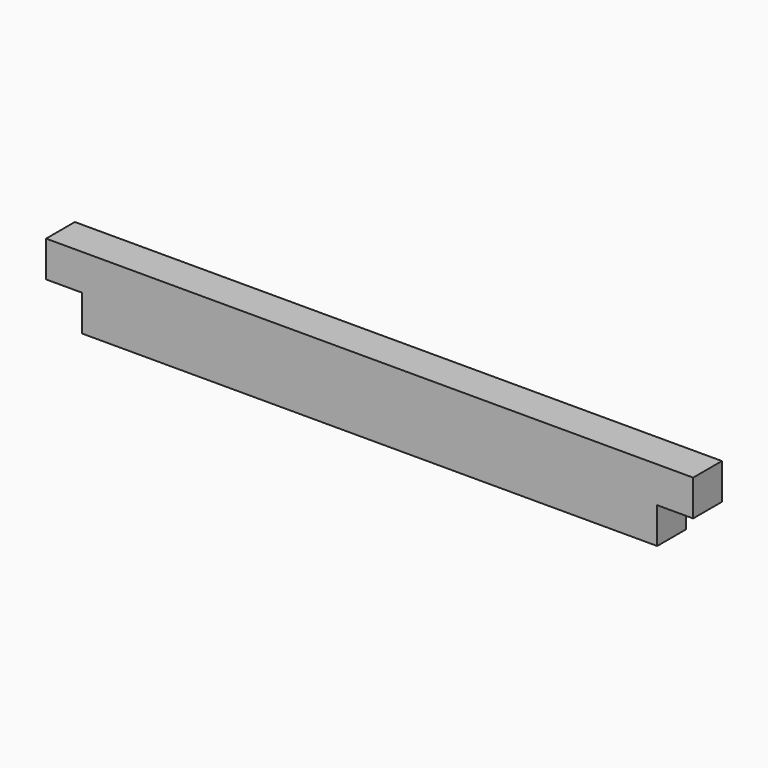
from build123d import *

# Parameters (mm, degrees)
F1_DEPTH = 3.175


# Not quite as in the source:
# - a length typed as a fraction of an inch, garbled in the dataset ("3 / 203.2 mm" for 3/8 in), is restored


with BuildPart() as f1:
    # F0 (on Front) → F1 (new body)
    with BuildSketch(Plane.XZ):
        Polygon((-24.5566335312, 3.175), (-24.5566335312, 0), (-21.3816335312, 0), (-21.3816335312, -3.175), (29.4183664688, -3.175), (29.4183664688, 0), (32.5933664688, 0), (32.5933664688, 3.175), align=None)
    extrude(amount=F1_DEPTH)


solid = f1.part
